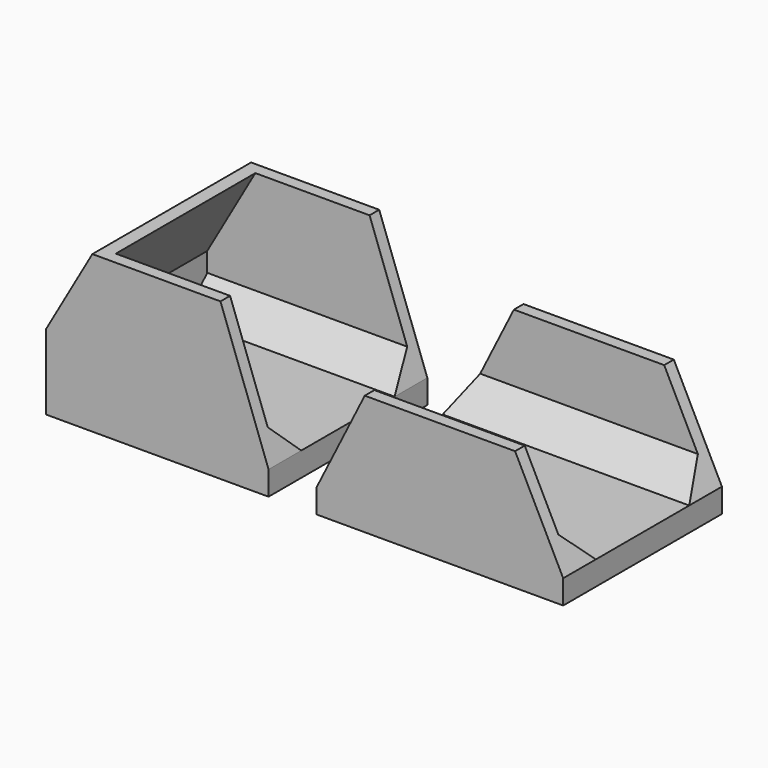
from build123d import *

# Parameters (mm, degrees)
F0_W      = 15.08125
F0_H      = 17.4625
F1_DEPTH  = 13.096875
F0_W_2    = 19.84375
F0_H_2    = 12.7
F2_DEPTH  = 11.509375
F3_SIZE   = 3.81
F3_2_SIZE = 3.81


# Not quite as in the source:
# - a feature names something its author has since deleted; it is built from what else it names


with BuildPart() as f1:
    # F0 (on Front) → F1 (new body, symmetric)
    with BuildSketch(Plane.XZ):
        Polygon((-25.4000246501, 0), (-19.0500246501, 0), (-19.0500246501, 17.4625), (-25.4000246501, 6.35), align=None)
        Polygon((-3.9687746501, 0), (2.3812253499, 0), (-3.9687746501, 17.4625), align=None)
        Polygon((-26.9875246501, -3.175), (-25.4000246501, -3.175), (-25.4000246501, 0), (-25.4000246501, 6.35), (-19.0500246501, 17.4625), (-20.8784295323, 17.4625), (-26.9875246501, 6.7715835439), (-26.9875246501, 6.35), align=None)
        with Locations((-11.5093996501, 8.73125)):
            Rectangle(F0_W, F0_H)
        Polygon((2.3812253499, -3.175), (2.3812253499, 0), (-3.9687746501, 0), (-19.0500246501, 0), (-25.4000246501, 0), (-25.4000246501, -3.175), align=None)
    extrude(amount=F1_DEPTH, both=True)


with BuildPart() as f1b:
    # F0 (on Front) → F1, piece 2 (new body, symmetric)
    with BuildSketch(Plane.XZ):
        Polygon((8.7312253499, 0), (15.0812253499, 0), (15.0812253499, 12.7), align=None)
        Polygon((34.9249753499, 0), (41.2749753499, 0), (34.9249753499, 12.7), align=None)
        Polygon((41.2749753499, -3.175), (41.2749753499, 0), (34.9249753499, 0), (15.0812253499, 0), (8.7312253499, 0), (8.7312253499, -3.175), align=None)
        with Locations((25.0031003499, 6.35)):
            Rectangle(F0_W_2, F0_H_2)
    extrude(amount=F1_DEPTH, both=True)


with BuildPart() as f2_tool:
    # F0 (on Front) → F2 (new body, symmetric)
    with BuildSketch(Plane.XZ):
        Polygon((-25.4000246501, 0), (-19.0500246501, 0), (-19.0500246501, 17.4625), (-25.4000246501, 6.35), align=None)
        with Locations((-11.5093996501, 8.73125)):
            Rectangle(F0_W, F0_H)
        Polygon((-3.9687746501, 0), (2.3812253499, 0), (-3.9687746501, 17.4625), align=None)
        with Locations((25.0031003499, 6.35)):
            Rectangle(F0_W_2, F0_H_2)
        Polygon((8.7312253499, 0), (15.0812253499, 0), (15.0812253499, 12.7), align=None)
        Polygon((34.9249753499, 0), (41.2749753499, 0), (34.9249753499, 12.7), align=None)
    extrude(amount=F2_DEPTH, both=True)


with BuildPart() as f1_1:
    add(f1.part)

    # F2: cut by f2_tool
    add(f2_tool.part, mode=Mode.SUBTRACT)

    # F3
    f3_edges = [f1_1.edges().sort_by_distance(p)[0] for p in [
        (-11.5094, -11.509375, 0),
        (-11.5094, 11.509375, 0),
    ]]
    chamfer(f3_edges, length=F3_SIZE)


with BuildPart() as f1b_1:
    add(f1b.part)

    # F2: cut by f2_tool
    add(f2_tool.part, mode=Mode.SUBTRACT)

    # F3#2
    f3_2_edges = [f1b_1.edges().sort_by_distance(p)[0] for p in [
        (25.0031, 11.509375, 0),
        (25.0031, -11.509375, 0),
    ]]
    chamfer(f3_2_edges, length=F3_2_SIZE)


solid = Compound([f1_1.part, f1b_1.part])
